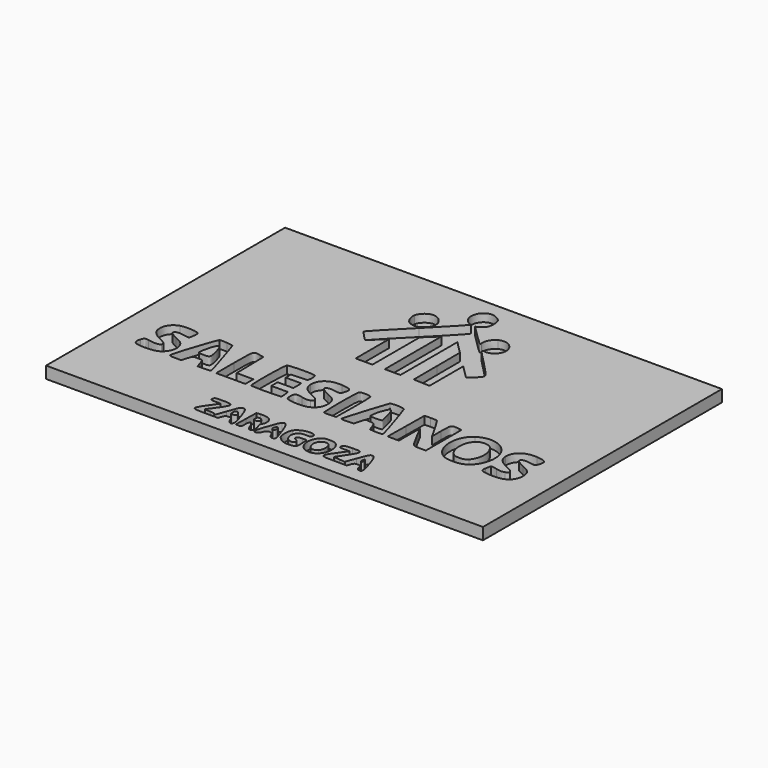
from build123d import *

# Parameters (mm, degrees)
F1_W     = 111
F1_H     = 75.8981681683
F2_DEPTH = 1
F0_W     = 111
F0_H     = 75.8981681683
F3_DEPTH = 3


# Not quite as in the source:
# - ends of sketch curves that miss each other by under 0.0002 mm in the source are joined
# - a feature names something its author has since deleted; it is built from what else it names


with BuildPart() as f2:
    # F1 (on Top) → F2 (new body)
    with BuildSketch(Plane.XY):
        Rectangle(F1_W, F1_H)
    extrude(amount=F2_DEPTH)

    # F0 (on Top) → F3 (join)
    with BuildSketch(Plane.XY):
        Rectangle(F0_W, F0_H)
        with BuildLine():
            add(Edge.make_bspline(
                [(-11.3553504545, -34.4155459636), (-11.5365297, -34.4751549818), (-11.8889547, -34.2324080727), (-12.1385170091, -33.8761071545)],
                knots=[0, 0, 0, 0, 1, 1, 1, 1], degree=3))
            add(Edge.make_bspline(
                [(-12.1385170091, -33.8761071545), (-12.3880803273, -33.5198062364), (-12.5922668455, -33.0645720273), (-12.5922668455, -32.8644723273)],
                knots=[0, 0, 0, 0, 1, 1, 1, 1], degree=3))
            add(Edge.make_bspline(
                [(-12.5922668455, -32.8644723273), (-12.5922668455, -32.6528175273), (-12.9379400182, -32.5006587273), (-13.4187698182, -32.5006587273)],
                knots=[0, 0, 0, 0, 1, 1, 1, 1], degree=3))
            add(Edge.make_bspline(
                [(-13.4187698182, -32.5006587273), (-14.0810664545, -32.5006587273), (-14.3044489091, -32.6704029545), (-14.5431100091, -33.3550216909)],
                knots=[0, 0, 0, 0, 1, 1, 1, 1], degree=3))
            Line((-14.5431100091, -33.3550216909), (-14.8409411727, -34.2093856636))
            Line((-14.8409411727, -34.2093856636), (-17.9884218545, -34.2093856636))
            add(Edge.make_bspline(
                [(-17.9884218545, -34.2093856636), (-21.7751353909, -34.2093856636), (-21.7852283182, -34.1913865091), (-19.6949197091, -31.1676597273)],
                knots=[0, 0, 0, 0, 1, 1, 1, 1], degree=3))
            Line((-19.6949197091, -31.1676597273), (-18.2539358727, -29.0832038455))
            Line((-18.2539358727, -29.0832038455), (-19.5723323182, -29.0832038455))
            add(Edge.make_bspline(
                [(-19.5723323182, -29.0832038455), (-20.7766661727, -29.0832038455), (-20.8828578545, -29.0277643909), (-20.7997259182, -28.4424311182)],
                knots=[0, 0, 0, 0, 1, 1, 1, 1], degree=3))
            add(Edge.make_bspline(
                [(-20.7997259182, -28.4424311182), (-20.7146050636, -27.8430916636), (-20.5708610727, -27.8016583909), (-18.5767137818, -27.8016583909)],
                knots=[0, 0, 0, 0, 1, 1, 1, 1], degree=3))
            add(Edge.make_bspline(
                [(-18.5767137818, -27.8016583909), (-15.8485941273, -27.8016583909), (-15.7638496636, -28.1012090455), (-17.7110812909, -30.8614874182)],
                knots=[0, 0, 0, 0, 1, 1, 1, 1], degree=3))
            Line((-17.7110812909, -30.8614874182), (-19.1687827364, -32.9278402091))
            Line((-19.1687827364, -32.9278402091), (-17.7316455545, -33.0139197))
            add(Edge.make_bspline(
                [(-17.7316455545, -33.0139197), (-16.6065747818, -33.0813098182), (-16.2931309636, -33.2049870273), (-16.2881591727, -33.5834960182)],
                knots=[0, 0, 0, 0, 1, 1, 1, 1], degree=3))
            add(Edge.make_bspline(
                [(-16.2881591727, -33.5834960182), (-16.2846556091, -33.8494197273), (-15.8040871636, -32.6572918364), (-15.2202039545, -30.9343246091)],
                knots=[0, 0, 0, 0, 1, 1, 1, 1], degree=3))
            add(Edge.make_bspline(
                [(-15.2202039545, -30.9343246091), (-14.2654788273, -28.1170437), (-14.0900635091, -27.8016583909), (-13.4778409909, -27.8016583909)],
                knots=[0, 0, 0, 0, 1, 1, 1, 1], degree=3))
            add(Edge.make_bspline(
                [(-13.4778409909, -27.8016583909), (-12.8766417818, -27.8016583909), (-12.6837490091, -28.1156794091), (-11.8273920818, -30.4885203545)],
                knots=[0, 0, 0, 0, 1, 1, 1, 1], degree=3))
            add(Edge.make_bspline(
                [(-11.8273920818, -30.4885203545), (-10.8589251545, -33.1719968182), (-10.7340208909, -34.2111253364), (-11.3553504545, -34.4155459636)],
                knots=[0, 0, 0, 0, 1, 1, 1, 1], degree=3))
        make_face(mode=Mode.SUBTRACT)
        with BuildLine():
            Line((-10.3326176455, -34.2093856636), (-10.2520942091, -31.0055220273))
            Line((-10.2520942091, -31.0055220273), (-10.1715697636, -27.8016583909))
            Line((-10.1715697636, -27.8016583909), (-9.2066033727, -27.7094779364))
            add(Edge.make_bspline(
                [(-9.2066033727, -27.7094779364), (-7.9795922182, -27.5922679909), (-7.0573345909, -27.8239118727), (-6.4892426455, -28.3920038182)],
                knots=[0, 0, 0, 0, 1, 1, 1, 1], degree=3))
            add(Edge.make_bspline(
                [(-6.4892426455, -28.3920038182), (-5.9702197636, -28.9110267), (-5.8971060818, -30.2481882), (-6.3623161636, -30.7133982818)],
                knots=[0, 0, 0, 0, 1, 1, 1, 1], degree=3))
            add(Edge.make_bspline(
                [(-6.3623161636, -30.7133982818), (-6.5993475818, -30.9504297), (-6.5993475818, -31.2720491727), (-6.3623161636, -31.9520028818)],
                knots=[0, 0, 0, 0, 1, 1, 1, 1], degree=3))
            add(Edge.make_bspline(
                [(-6.3623161636, -31.9520028818), (-6.1862227364, -32.4571426909), (-6.0421457455, -33.1717041818), (-6.0421457455, -33.5399123727)],
                knots=[0, 0, 0, 0, 1, 1, 1, 1], degree=3))
            add(Edge.make_bspline(
                [(-6.0421457455, -33.5399123727), (-6.0421457455, -34.5283562727), (-7.1124894818, -34.4433070636), (-7.4729629909, -33.4262191091)],
                knots=[0, 0, 0, 0, 1, 1, 1, 1], degree=3))
            add(Edge.make_bspline(
                [(-7.4729629909, -33.4262191091), (-8.2103047091, -31.3457925273), (-8.8900243091, -31.0953492818), (-8.8900243091, -32.9041084091)],
                knots=[0, 0, 0, 0, 1, 1, 1, 1], degree=3))
            add(Edge.make_bspline(
                [(-8.8900243091, -32.9041084091), (-8.8900243091, -34.1110457182), (-8.9443678909, -34.2093856636), (-9.6113214818, -34.2093856636)],
                knots=[0, 0, 0, 0, 1, 1, 1, 1], degree=3))
            Line((-9.6113214818, -34.2093856636), (-10.3326176455, -34.2093856636))
        make_face(mode=Mode.SUBTRACT)
        with BuildLine():
            add(Edge.make_bspline(
                [(-4.081359, -33.3264916636), (-4.3966989, -34.2310780909), (-5.4122066182, -34.6980611455), (-5.6599636636, -34.0524185455)],
                knots=[0, 0, 0, 0, 1, 1, 1, 1], degree=3))
            add(Edge.make_bspline(
                [(-5.6599636636, -34.0524185455), (-5.8610835545, -33.5283068182), (-4.0886718818, -28.3318135636), (-3.5587952182, -27.8920557818)],
                knots=[0, 0, 0, 0, 1, 1, 1, 1], degree=3))
            add(Edge.make_bspline(
                [(-3.5587952182, -27.8920557818), (-2.8344657273, -27.2909140909), (-2.2841247, -28.0040457), (-1.3082682, -30.8082861273)],
                knots=[0, 0, 0, 0, 1, 1, 1, 1], degree=3))
            add(Edge.make_bspline(
                [(-1.3082682, -30.8082861273), (-0.1767432818, -34.0598515091), (-0.1645312636, -34.2093856636), (-1.0304967545, -34.2093856636)],
                knots=[0, 0, 0, 0, 1, 1, 1, 1], degree=3))
            add(Edge.make_bspline(
                [(-1.0304967545, -34.2093856636), (-1.5345770182, -34.2093856636), (-1.7929880455, -33.9845511273), (-2.0124431182, -33.3550216909)],
                knots=[0, 0, 0, 0, 1, 1, 1, 1], degree=3))
            add(Edge.make_bspline(
                [(-2.0124431182, -33.3550216909), (-2.4296568, -32.1581974909), (-3.6681342545, -32.1411196364), (-4.081359, -33.3264916636)],
                knots=[0, 0, 0, 0, 1, 1, 1, 1], degree=3))
        make_face(mode=Mode.SUBTRACT)
        with BuildLine():
            add(Edge.make_bspline(
                [(-42.0060337364, -19.2096196364), (-42.9500251636, -19.6575712364), (-45.3833419364, -19.7937904364), (-46.9597225636, -19.4869289182)],
                knots=[0, 0, 0, 0, 1, 1, 1, 1], degree=3))
            add(Edge.make_bspline(
                [(-46.9597225636, -19.4869289182), (-48.0138643364, -19.2817272545), (-48.2886367636, -18.7088058), (-47.8990519909, -17.5283510727)],
                knots=[0, 0, 0, 0, 1, 1, 1, 1], degree=3))
            add(Edge.make_bspline(
                [(-47.8990519909, -17.5283510727), (-47.5662205091, -16.5198636), (-47.5247781545, -16.4950984909), (-46.5205853727, -16.7045686091)],
                knots=[0, 0, 0, 0, 1, 1, 1, 1], degree=3))
            add(Edge.make_bspline(
                [(-46.5205853727, -16.7045686091), (-44.9145808636, -17.0395756909), (-43.6095346909, -16.9735105091), (-43.3439328818, -16.5437598818)],
                knots=[0, 0, 0, 0, 1, 1, 1, 1], degree=3))
            add(Edge.make_bspline(
                [(-43.3439328818, -16.5437598818), (-42.9966027818, -15.9817648636), (-43.1955238636, -15.7840284545), (-45.0498979364, -14.8479422455)],
                knots=[0, 0, 0, 0, 1, 1, 1, 1], degree=3))
            add(Edge.make_bspline(
                [(-45.0498979364, -14.8479422455), (-47.1731503364, -13.7761282636), (-47.9059642636, -12.8574286909), (-47.9059642636, -11.2674061636)],
                knots=[0, 0, 0, 0, 1, 1, 1, 1], degree=3))
            add(Edge.make_bspline(
                [(-47.9059642636, -11.2674061636), (-47.9059642636, -9.7685731636), (-46.9405306636, -8.4891811091), (-45.4344271636, -7.9921210909)],
                knots=[0, 0, 0, 0, 1, 1, 1, 1], degree=3))
            add(Edge.make_bspline(
                [(-45.4344271636, -7.9921210909), (-44.3034774273, -7.6188755182), (-41.1813158455, -7.7847246545), (-40.7236820182, -8.2423584818)],
                knots=[0, 0, 0, 0, 1, 1, 1, 1], degree=3))
            add(Edge.make_bspline(
                [(-40.7236820182, -8.2423584818), (-40.5603879, -8.4056526), (-40.5263724545, -9.0221476091), (-40.6426772455, -9.7105423636)],
                knots=[0, 0, 0, 0, 1, 1, 1, 1], degree=3))
            Line((-40.6426772455, -9.7105423636), (-40.8431644364, -10.8972302455))
            Line((-40.8431644364, -10.8972302455), (-42.0250662, -10.6883585182))
            add(Edge.make_bspline(
                [(-42.0250662, -10.6883585182), (-43.4975901818, -10.4281250727), (-44.2100093727, -10.4643645545), (-44.5631094545, -10.8174646364)],
                knots=[0, 0, 0, 0, 1, 1, 1, 1], degree=3))
            add(Edge.make_bspline(
                [(-44.5631094545, -10.8174646364), (-44.9928943909, -11.2472495727), (-44.5569015273, -11.6855572909), (-42.9671898, -12.4218283636)],
                knots=[0, 0, 0, 0, 1, 1, 1, 1], degree=3))
            add(Edge.make_bspline(
                [(-42.9671898, -12.4218283636), (-42.1592662091, -12.7960164273), (-41.2948981091, -13.2697704818), (-41.0463751636, -13.4746119)],
                knots=[0, 0, 0, 0, 1, 1, 1, 1], degree=3))
            add(Edge.make_bspline(
                [(-41.0463751636, -13.4746119), (-39.2149609364, -14.9841271364), (-39.7422745091, -18.1353939273), (-42.0060337364, -19.2096196364)],
                knots=[0, 0, 0, 0, 1, 1, 1, 1], degree=3))
        make_face(mode=Mode.SUBTRACT)
        with BuildLine():
            add(Edge.make_bspline(
                [(-37.5612062455, -19.4004155182), (-38.7397729636, -19.4004155182), (-39.0775399091, -19.3022632636), (-39.0775399091, -18.9597838636)],
                knots=[0, 0, 0, 0, 1, 1, 1, 1], degree=3))
            add(Edge.make_bspline(
                [(-39.0775399091, -18.9597838636), (-39.0775399091, -17.9400753), (-35.8349251636, -8.0276481545), (-35.4534686182, -7.8812704364)],
                knots=[0, 0, 0, 0, 1, 1, 1, 1], degree=3))
            add(Edge.make_bspline(
                [(-35.4534686182, -7.8812704364), (-35.2287682909, -7.7950416), (-34.3552104, -7.8055563273), (-33.5122289727, -7.9046228182)],
                knots=[0, 0, 0, 0, 1, 1, 1, 1], degree=3))
            Line((-33.5122289727, -7.9046228182), (-31.9795349182, -8.0847596727))
            Line((-31.9795349182, -8.0847596727), (-31.1347462091, -10.6811142545))
            add(Edge.make_bspline(
                [(-31.1347462091, -10.6811142545), (-29.9778497182, -14.2366844182), (-28.5403886182, -18.9568383273), (-28.5403886182, -19.2001442727)],
                knots=[0, 0, 0, 0, 1, 1, 1, 1], degree=3))
            add(Edge.make_bspline(
                [(-28.5403886182, -19.2001442727), (-28.5403886182, -19.3102946182), (-29.2868141727, -19.4004155182), (-30.1991151, -19.4004155182)],
                knots=[0, 0, 0, 0, 1, 1, 1, 1], degree=3))
            Line((-30.1991151, -19.4004155182), (-31.8578456182, -19.4004155182))
            Line((-31.8578456182, -19.4004155182), (-32.2779412636, -18.0476736545))
            add(Edge.make_bspline(
                [(-32.2779412636, -18.0476736545), (-32.6957079273, -16.7024323636), (-32.7049865182, -16.6949307818), (-33.9513580909, -16.6949307818)],
                knots=[0, 0, 0, 0, 1, 1, 1, 1], degree=3))
            add(Edge.make_bspline(
                [(-33.9513580909, -16.6949307818), (-35.1977296636, -16.6949307818), (-35.2070072455, -16.7024212636), (-35.6247739091, -18.0476736545)],
                knots=[0, 0, 0, 0, 1, 1, 1, 1], degree=3))
            Line((-35.6247739091, -18.0476736545), (-36.0448735909, -19.4004155182))
            Line((-36.0448735909, -19.4004155182), (-37.5612062455, -19.4004155182))
        make_face(mode=Mode.SUBTRACT)
        with BuildLine():
            Line((-27.1164493364, -19.4004155182), (-27.1164493364, -13.6957218818))
            add(Edge.make_bspline(
                [(-27.1164493364, -13.6957218818), (-27.1164493364, -7.3469991818), (-27.1530157636, -7.4570899909), (-25.1976417818, -7.9189509)],
                knots=[0, 0, 0, 0, 1, 1, 1, 1], degree=3))
            Line((-25.1976417818, -7.9189509), (-24.1261759364, -8.1720329182))
            Line((-24.1261759364, -8.1720329182), (-24.0475606909, -12.5046787636))
            Line((-24.0475606909, -12.5046787636), (-23.9689474636, -16.8373246091))
            Line((-23.9689474636, -16.8373246091), (-21.8404548545, -16.8373246091))
            Line((-21.8404548545, -16.8373246091), (-19.7119642636, -16.8373246091))
            Line((-19.7119642636, -16.8373246091), (-19.7119642636, -18.1188700636))
            Line((-19.7119642636, -18.1188700636), (-19.7119642636, -19.4004155182))
            Line((-19.7119642636, -19.4004155182), (-23.4142068, -19.4004155182))
            Line((-23.4142068, -19.4004155182), (-27.1164493364, -19.4004155182))
        make_face(mode=Mode.SUBTRACT)
        with BuildLine():
            add(Edge.make_bspline(
                [(-10.7686448182, -19.1601116182), (-10.9430429727, -19.4422968273), (-18.1037811273, -19.4897362091), (-18.3829582364, -19.2105560727)],
                knots=[0, 0, 0, 0, 1, 1, 1, 1], degree=3))
            add(Edge.make_bspline(
                [(-18.3829582364, -19.2105560727), (-18.7421582727, -18.8513530091), (-18.6001973455, -8.4349888909), (-18.2310668455, -8.0658583909)],
                knots=[0, 0, 0, 0, 1, 1, 1, 1], degree=3))
            add(Edge.make_bspline(
                [(-18.2310668455, -8.0658583909), (-17.8347907909, -7.6695813273), (-11.8234596545, -7.5882970364), (-11.2198174364, -7.9710522818)],
                knots=[0, 0, 0, 0, 1, 1, 1, 1], degree=3))
            add(Edge.make_bspline(
                [(-11.2198174364, -7.9710522818), (-10.9844086364, -8.1203180182), (-10.8780686182, -8.6238089727), (-10.9350297818, -9.3194348727)],
                knots=[0, 0, 0, 0, 1, 1, 1, 1], degree=3))
            Line((-10.9350297818, -9.3194348727), (-11.0259337364, -10.4295973364))
            Line((-11.0259337364, -10.4295973364), (-13.0906457455, -10.5132711545))
            Line((-13.0906457455, -10.5132711545), (-15.1553577545, -10.5969449727))
            Line((-15.1553577545, -10.5969449727), (-15.1553577545, -11.4388315364))
            Line((-15.1553577545, -11.4388315364), (-15.1553577545, -12.2807191091))
            Line((-15.1553577545, -12.2807191091), (-13.1618431636, -12.2807191091))
            Line((-13.1618431636, -12.2807191091), (-11.1683275636, -12.2807191091))
            Line((-11.1683275636, -12.2807191091), (-11.1683275636, -13.5622645636))
            Line((-11.1683275636, -13.5622645636), (-11.1683275636, -14.8438100182))
            Line((-11.1683275636, -14.8438100182), (-13.1618431636, -14.8438100182))
            Line((-13.1618431636, -14.8438100182), (-15.1553577545, -14.8438100182))
            Line((-15.1553577545, -14.8438100182), (-15.1553577545, -15.8405678182))
            Line((-15.1553577545, -15.8405678182), (-15.1553577545, -16.8373246091))
            Line((-15.1553577545, -16.8373246091), (-13.0567100182, -16.8373246091))
            Line((-13.0567100182, -16.8373246091), (-10.9580632909, -16.8373246091))
            Line((-10.9580632909, -16.8373246091), (-10.7890930364, -17.8785661636))
            add(Edge.make_bspline(
                [(-10.7890930364, -17.8785661636), (-10.6961608091, -18.4512525), (-10.6869568909, -19.0279479545), (-10.7686448182, -19.1601116182)],
                knots=[0, 0, 0, 0, 1, 1, 1, 1], degree=3))
        make_face(mode=Mode.SUBTRACT)
        with BuildLine():
            add(Edge.make_bspline(
                [(-3.6601170273, -19.2925326), (-4.7367383182, -19.7423722091), (-7.5199381909, -19.7765894727), (-8.6764340727, -19.3542001636)],
                knots=[0, 0, 0, 0, 1, 1, 1, 1], degree=3))
            add(Edge.make_bspline(
                [(-8.6764340727, -19.3542001636), (-9.30735, -19.1237702182), (-9.4587519818, -18.8928438), (-9.4552403455, -18.1663356818)],
                knots=[0, 0, 0, 0, 1, 1, 1, 1], degree=3))
            add(Edge.make_bspline(
                [(-9.4552403455, -18.1663356818), (-9.4476075818, -16.5868480636), (-9.1572386455, -16.3974639), (-7.3923336, -16.8208582636)],
                knots=[0, 0, 0, 0, 1, 1, 1, 1], degree=3))
            add(Edge.make_bspline(
                [(-7.3923336, -16.8208582636), (-6.2100685636, -17.1044784), (-5.7048712364, -17.1140647636), (-5.233539, -16.8618142364)],
                knots=[0, 0, 0, 0, 1, 1, 1, 1], degree=3))
            add(Edge.make_bspline(
                [(-5.233539, -16.8618142364), (-4.1449115455, -16.2791974364), (-4.5131762455, -15.7128340636), (-6.5470978636, -14.8416566182)],
                knots=[0, 0, 0, 0, 1, 1, 1, 1], degree=3))
            add(Edge.make_bspline(
                [(-6.5470978636, -14.8416566182), (-8.4610315091, -14.0218752), (-9.4599507818, -12.8670059727), (-9.4585350273, -11.4757006909)],
                knots=[0, 0, 0, 0, 1, 1, 1, 1], degree=3))
            add(Edge.make_bspline(
                [(-9.4585350273, -11.4757006909), (-9.4559719364, -9.0022039364), (-7.4633342455, -7.5549122727), (-4.3989229364, -7.8008943273)],
                knots=[0, 0, 0, 0, 1, 1, 1, 1], degree=3))
            add(Edge.make_bspline(
                [(-4.3989229364, -7.8008943273), (-2.0766848727, -7.9873026818), (-1.6656619636, -8.3485249364), (-2.1139102364, -9.8090538545)],
                knots=[0, 0, 0, 0, 1, 1, 1, 1], degree=3))
            add(Edge.make_bspline(
                [(-2.1139102364, -9.8090538545), (-2.4429707455, -10.8812260636), (-2.4537276545, -10.8875480182), (-3.6029833091, -10.6842545455)],
                knots=[0, 0, 0, 0, 1, 1, 1, 1], degree=3))
            add(Edge.make_bspline(
                [(-3.6029833091, -10.6842545455), (-5.0516140364, -10.4280090273), (-5.7650988273, -10.4658166364), (-6.1167458182, -10.8174646364)],
                knots=[0, 0, 0, 0, 1, 1, 1, 1], degree=3))
            add(Edge.make_bspline(
                [(-6.1167458182, -10.8174646364), (-6.5633442273, -11.2640630455), (-6.1060383545, -11.6764986818), (-4.2121048909, -12.5352542182)],
                knots=[0, 0, 0, 0, 1, 1, 1, 1], degree=3))
            add(Edge.make_bspline(
                [(-4.2121048909, -12.5352542182), (-2.0595777545, -13.511253), (-1.4855402455, -14.2423746818), (-1.4855402455, -16.0079225182)],
                knots=[0, 0, 0, 0, 1, 1, 1, 1], degree=3))
            add(Edge.make_bspline(
                [(-1.4855402455, -16.0079225182), (-1.4855402455, -17.5672424455), (-2.2329970909, -18.6962436273), (-3.6601170273, -19.2925326)],
                knots=[0, 0, 0, 0, 1, 1, 1, 1], degree=3))
        make_face(mode=Mode.SUBTRACT)
        with BuildLine():
            add(Edge.make_bspline(
                [(4.8672834, -33.9506840182), (4.3306034455, -34.4865778909), (2.3567782364, -34.5194823273), (1.3663000091, -34.0090458)],
                knots=[0, 0, 0, 0, 1, 1, 1, 1], degree=3))
            add(Edge.make_bspline(
                [(1.3663000091, -34.0090458), (0.8202627545, -33.7276497), (0.2134197, -33.1770291545), (0.0177559636, -32.7854463818)],
                knots=[0, 0, 0, 0, 1, 1, 1, 1], degree=3))
            add(Edge.make_bspline(
                [(0.0177559636, -32.7854463818), (-0.4760325818, -31.7972123727), (-0.4342824545, -29.9049994091), (0.0980806091, -29.1449430545)],
                knots=[0, 0, 0, 0, 1, 1, 1, 1], degree=3))
            add(Edge.make_bspline(
                [(0.0980806091, -29.1449430545), (1.2483695727, -27.5026798909), (4.7797932, -27.0494568), (4.7797932, -28.5440970273)],
                knots=[0, 0, 0, 0, 1, 1, 1, 1], degree=3))
            add(Edge.make_bspline(
                [(4.7797932, -28.5440970273), (4.7797932, -29.0003413364), (4.5634148455, -29.0832038455), (3.3720013909, -29.0832038455)],
                knots=[0, 0, 0, 0, 1, 1, 1, 1], degree=3))
            add(Edge.make_bspline(
                [(3.3720013909, -29.0832038455), (2.2400728364, -29.0832038455), (1.8773409818, -29.2072312091), (1.5208806273, -29.7161480455)],
                knots=[0, 0, 0, 0, 1, 1, 1, 1], degree=3))
            add(Edge.make_bspline(
                [(1.5208806273, -29.7161480455), (0.5511694909, -31.1006036182), (1.3778712545, -33.0702340364), (2.9286724364, -33.0702340364)],
                knots=[0, 0, 0, 0, 1, 1, 1, 1], degree=3))
            add(Edge.make_bspline(
                [(2.9286724364, -33.0702340364), (3.8298380455, -33.0702340364), (3.9254443636, -32.0719898455), (3.0462981273, -31.8420886636)],
                knots=[0, 0, 0, 0, 1, 1, 1, 1], degree=3))
            add(Edge.make_bspline(
                [(3.0462981273, -31.8420886636), (2.6611281273, -31.7413652455), (2.4871003091, -31.5041572364), (2.5518183545, -31.1681017091)],
                knots=[0, 0, 0, 0, 1, 1, 1, 1], degree=3))
            add(Edge.make_bspline(
                [(2.5518183545, -31.1681017091), (2.6284921091, -30.7699679182), (2.9153332636, -30.6495369545), (3.7869375545, -30.6495369545)],
                knots=[0, 0, 0, 0, 1, 1, 1, 1], degree=3))
            Line((3.7869375545, -30.6495369545), (4.9221870273, -30.6495369545))
            Line((4.9221870273, -30.6495369545), (5.0096772273, -32.185338))
            add(Edge.make_bspline(
                [(5.0096772273, -32.185338), (5.0577977455, -33.0300278182), (4.9937295545, -33.8244346364), (4.8672834, -33.9506840182)],
                knots=[0, 0, 0, 0, 1, 1, 1, 1], degree=3))
        make_face(mode=Mode.SUBTRACT)
        with BuildLine():
            add(Edge.make_bspline(
                [(10.5467477455, -33.3512365909), (9.5478718636, -34.4475502909), (8.3566612364, -34.6719065182), (7.0651621091, -34.0069670727)],
                knots=[0, 0, 0, 0, 1, 1, 1, 1], degree=3))
            add(Edge.make_bspline(
                [(7.0651621091, -34.0069670727), (5.2252079455, -33.0596517), (4.8539926636, -30.3067487727), (6.3341625273, -28.5859470545)],
                knots=[0, 0, 0, 0, 1, 1, 1, 1], degree=3))
            add(Edge.make_bspline(
                [(6.3341625273, -28.5859470545), (6.9086258727, -27.9180963818), (7.2275056636, -27.8016583909), (8.4820357364, -27.8016583909)],
                knots=[0, 0, 0, 0, 1, 1, 1, 1], degree=3))
            add(Edge.make_bspline(
                [(8.4820357364, -27.8016583909), (9.7431531545, -27.8016583909), (10.0542589091, -27.9167149364), (10.6426023, -28.6007050091)],
                knots=[0, 0, 0, 0, 1, 1, 1, 1], degree=3))
            add(Edge.make_bspline(
                [(10.6426023, -28.6007050091), (11.6729164091, -29.7985171091), (11.6251117364, -32.1676789091), (10.5467477455, -33.3512365909)],
                knots=[0, 0, 0, 0, 1, 1, 1, 1], degree=3))
        make_face(mode=Mode.SUBTRACT)
        with BuildLine():
            add(Edge.make_bspline(
                [(21.0134291727, -30.9365718545), (21.9769263273, -33.9176635364), (21.9674196818, -34.5173410364), (20.9603439273, -34.285347)],
                knots=[0, 0, 0, 0, 1, 1, 1, 1], degree=3))
            add(Edge.make_bspline(
                [(20.9603439273, -34.285347), (20.6965968273, -34.2245876182), (20.3980673727, -33.7981770818), (20.2969423364, -33.3377662364)],
                knots=[0, 0, 0, 0, 1, 1, 1, 1], degree=3))
            add(Edge.make_bspline(
                [(20.2969423364, -33.3377662364), (20.1464576182, -32.6526126818), (19.9671613364, -32.5006587273), (19.3092068182, -32.5006587273)],
                knots=[0, 0, 0, 0, 1, 1, 1, 1], degree=3))
            add(Edge.make_bspline(
                [(19.3092068182, -32.5006587273), (18.6720537, -32.5006587273), (18.4435602, -32.6778530727), (18.2074965, -33.3550216909)],
                knots=[0, 0, 0, 0, 1, 1, 1, 1], degree=3))
            Line((18.2074965, -33.3550216909), (17.9096653364, -34.2093856636))
            Line((17.9096653364, -34.2093856636), (14.7621836455, -34.2093856636))
            add(Edge.make_bspline(
                [(14.7621836455, -34.2093856636), (10.9602399, -34.2093856636), (10.9236623727, -34.1435656909), (13.0460610818, -31.1213818091)],
                knots=[0, 0, 0, 0, 1, 1, 1, 1], degree=3))
            Line((13.0460610818, -31.1213818091), (14.4774161727, -29.0832038455))
            Line((14.4774161727, -29.0832038455), (13.1686444364, -29.0832038455))
            add(Edge.make_bspline(
                [(13.1686444364, -29.0832038455), (11.9742985636, -29.0832038455), (11.8678334182, -29.0271831545), (11.9508805909, -28.4424311182)],
                knots=[0, 0, 0, 0, 1, 1, 1, 1], degree=3))
            add(Edge.make_bspline(
                [(11.9508805909, -28.4424311182), (12.0344091, -27.8542986273), (12.2118426, -27.7947774), (14.1107145545, -27.7179018273)],
                knots=[0, 0, 0, 0, 1, 1, 1, 1], degree=3))
            add(Edge.make_bspline(
                [(14.1107145545, -27.7179018273), (16.8515013273, -27.6069401727), (16.9430692636, -27.8948156455), (15.0684134727, -30.7287142636)],
                knots=[0, 0, 0, 0, 1, 1, 1, 1], degree=3))
            Line((15.0684134727, -30.7287142636), (13.6136686636, -32.9278402091))
            Line((13.6136686636, -32.9278402091), (15.1060798091, -33.0702340364))
            Line((15.1060798091, -33.0702340364), (16.5984909545, -33.2126278636))
            Line((16.5984909545, -33.2126278636), (17.5364308636, -30.6513967091))
            add(Edge.make_bspline(
                [(17.5364308636, -30.6513967091), (18.5974334455, -27.7541160818), (18.7475770909, -27.5346751364), (19.5045516818, -27.7749306)],
                knots=[0, 0, 0, 0, 1, 1, 1, 1], degree=3))
            add(Edge.make_bspline(
                [(19.5045516818, -27.7749306), (19.8976127727, -27.8996824909), (20.3136478364, -28.7714240182), (21.0134291727, -30.9365718545)],
                knots=[0, 0, 0, 0, 1, 1, 1, 1], degree=3))
        make_face(mode=Mode.SUBTRACT)
        with BuildLine():
            add(Edge.make_bspline(
                [(1.7785822636, -19.3420113545), (0.9893974909, -19.3882065273), (0.2525088545, -19.3348064455), (0.1410517364, -19.2233493273)],
                knots=[0, 0, 0, 0, 1, 1, 1, 1], degree=3))
            add(Edge.make_bspline(
                [(0.1410517364, -19.2233493273), (0.0295915909, -19.1118912), (-0.0615999545, -16.6228140818), (-0.0615999545, -13.6920649364)],
                knots=[0, 0, 0, 0, 1, 1, 1, 1], degree=3))
            add(Edge.make_bspline(
                [(-0.0615999545, -13.6920649364), (-0.0615999545, -9.7551855545), (0.0320830364, -8.2856807727), (0.2970844364, -8.0657473909)],
                knots=[0, 0, 0, 0, 1, 1, 1, 1], degree=3))
            add(Edge.make_bspline(
                [(0.2970844364, -8.0657473909), (0.7040830909, -7.7279683364), (2.7342337364, -7.8429401182), (3.1167235909, -8.2254309818)],
                knots=[0, 0, 0, 0, 1, 1, 1, 1], degree=3))
            add(Edge.make_bspline(
                [(3.1167235909, -8.2254309818), (3.2553605727, -8.3640679636), (3.3338426182, -10.9031172818), (3.2911278, -13.8677617909)],
                knots=[0, 0, 0, 0, 1, 1, 1, 1], degree=3))
            Line((3.2911278, -13.8677617909), (3.2134600909, -19.2580216909))
            Line((3.2134600909, -19.2580216909), (1.7785822636, -19.3420113545))
        make_face(mode=Mode.SUBTRACT)
        with BuildLine():
            add(Edge.make_bspline(
                [(6.1039061455, -19.3434301364), (5.2070665091, -19.3910410636), (4.4950055455, -19.3079000455), (4.4950055455, -19.1555777727)],
                knots=[0, 0, 0, 0, 1, 1, 1, 1], degree=3))
            add(Edge.make_bspline(
                [(4.4950055455, -19.1555777727), (4.4950055455, -18.6306850091), (7.6846783364, -8.4332744455), (7.9500460364, -8.1097810909)],
                knots=[0, 0, 0, 0, 1, 1, 1, 1], degree=3))
            add(Edge.make_bspline(
                [(7.9500460364, -8.1097810909), (8.2585745727, -7.7336787818), (11.2335340091, -7.7926096909), (11.6059107545, -8.1821995091)],
                knots=[0, 0, 0, 0, 1, 1, 1, 1], degree=3))
            add(Edge.make_bspline(
                [(11.6059107545, -8.1821995091), (11.8817316273, -8.4707722636), (15.0321568364, -18.4605109091), (15.0321568364, -19.0465444909)],
                knots=[0, 0, 0, 0, 1, 1, 1, 1], degree=3))
            add(Edge.make_bspline(
                [(15.0321568364, -19.0465444909), (15.0321568364, -19.3311979364), (14.6233297091, -19.4070260727), (13.4314581273, -19.3434301364)],
                knots=[0, 0, 0, 0, 1, 1, 1, 1], degree=3))
            Line((13.4314581273, -19.3434301364), (11.8307624455, -19.2580216909))
            Line((11.8307624455, -19.2580216909), (11.3602304182, -17.9764762364))
            add(Edge.make_bspline(
                [(11.3602304182, -17.9764762364), (10.9151184, -16.7641624909), (10.8253789364, -16.6902344727), (9.6990710182, -16.6080056727)],
                knots=[0, 0, 0, 0, 1, 1, 1, 1], degree=3))
            Line((9.6990710182, -16.6080056727), (8.5084446545, -16.5210795545))
            Line((8.5084446545, -16.5210795545), (8.1106267091, -17.8895511273))
            Line((8.1106267091, -17.8895511273), (7.7128097727, -19.2580216909))
            Line((7.7128097727, -19.2580216909), (6.1039061455, -19.3434301364))
        make_face(mode=Mode.SUBTRACT)
        with BuildLine():
            Line((16.4443149818, -19.4004155182), (16.5214065, -13.6382824091))
            Line((16.5214065, -13.6382824091), (16.5984909545, -7.8761472818))
            Line((16.5984909545, -7.8761472818), (18.0792622364, -7.8456434727))
            add(Edge.make_bspline(
                [(18.0792622364, -7.8456434727), (18.8936874, -7.8288693545), (19.6720809545, -7.8907730455), (19.8090267, -7.9832158636)],
                knots=[0, 0, 0, 0, 1, 1, 1, 1], degree=3))
            add(Edge.make_bspline(
                [(19.8090267, -7.9832158636), (19.9459694182, -8.0756607), (20.7842232545, -9.4328405455), (21.6718095273, -10.9991736545)],
                knots=[0, 0, 0, 0, 1, 1, 1, 1], degree=3))
            Line((21.6718095273, -10.9991736545), (23.2856001818, -13.8470522182))
            Line((23.2856001818, -13.8470522182), (23.2881632727, -10.9477836818))
            add(Edge.make_bspline(
                [(23.2881632727, -10.9477836818), (23.2911542182, -7.7511764182), (23.3304340909, -7.6945401818), (25.3555786364, -7.9678514455)],
                knots=[0, 0, 0, 0, 1, 1, 1, 1], degree=3))
            Line((25.3555786364, -7.9678514455), (26.1387451909, -8.0735476636))
            Line((26.1387451909, -8.0735476636), (26.1387451909, -13.7369815909))
            Line((26.1387451909, -13.7369815909), (26.1387451909, -19.4004155182))
            Line((26.1387451909, -19.4004155182), (24.6072812182, -19.4004155182))
            add(Edge.make_bspline(
                [(24.6072812182, -19.4004155182), (23.7274770545, -19.4004155182), (22.9517525455, -19.2489398727), (22.7842454727, -19.0444314545)],
                knots=[0, 0, 0, 0, 1, 1, 1, 1], degree=3))
            add(Edge.make_bspline(
                [(22.7842454727, -19.0444314545), (22.6238787273, -18.8486395636), (21.7771243091, -17.3428236545), (20.9025724636, -15.6981729818)],
                knots=[0, 0, 0, 0, 1, 1, 1, 1], degree=3))
            Line((20.9025724636, -15.6981729818), (19.3124732455, -12.7079005909))
            Line((19.3124732455, -12.7079005909), (19.3081442455, -16.0541580545))
            Line((19.3081442455, -16.0541580545), (19.3039867909, -19.4004155182))
            Line((19.3039867909, -19.4004155182), (17.8741493727, -19.4004155182))
            Line((17.8741493727, -19.4004155182), (16.4443149818, -19.4004155182))
        make_face(mode=Mode.SUBTRACT)
        with BuildLine():
            add(Edge.make_bspline(
                [(35.6216770091, -19.3004438727), (34.4609469818, -19.7854260818), (31.9589060727, -19.7791011), (30.8325900818, -19.2883408364)],
                knots=[0, 0, 0, 0, 1, 1, 1, 1], degree=3))
            add(Edge.make_bspline(
                [(30.8325900818, -19.2883408364), (27.0607687091, -17.6448435545), (26.5969057636, -11.0224543909), (30.0916206818, -8.7097603091)],
                knots=[0, 0, 0, 0, 1, 1, 1, 1], degree=3))
            add(Edge.make_bspline(
                [(30.0916206818, -8.7097603091), (33.0660140182, -6.7414013455), (36.9778659273, -7.8151790182), (38.4232150909, -10.9967296364)],
                knots=[0, 0, 0, 0, 1, 1, 1, 1], degree=3))
            add(Edge.make_bspline(
                [(38.4232150909, -10.9967296364), (39.7858823727, -13.9962866727), (38.3860331182, -18.1454212636), (35.6216770091, -19.3004438727)],
                knots=[0, 0, 0, 0, 1, 1, 1, 1], degree=3))
        make_face(mode=Mode.SUBTRACT)
        with BuildLine():
            add(Edge.make_bspline(
                [(45.8929732091, -19.2925326), (44.8046908636, -19.7472451091), (42.0304184182, -19.7751141818), (40.8438102545, -19.3432505182)],
                knots=[0, 0, 0, 0, 1, 1, 1, 1], degree=3))
            add(Edge.make_bspline(
                [(40.8438102545, -19.3432505182), (40.0911525545, -19.0693247182), (40.0395456273, -18.9586900091), (40.1790948273, -17.9182738909)],
                knots=[0, 0, 0, 0, 1, 1, 1, 1], degree=3))
            add(Edge.make_bspline(
                [(40.1790948273, -17.9182738909), (40.2623074909, -17.2978807636), (40.4075237455, -16.7131489091), (40.5018021, -16.6188725727)],
                knots=[0, 0, 0, 0, 1, 1, 1, 1], degree=3))
            add(Edge.make_bspline(
                [(40.5018021, -16.6188725727), (40.5960784364, -16.5245962364), (41.2881129818, -16.6050601364), (42.0396566455, -16.7976683455)],
                knots=[0, 0, 0, 0, 1, 1, 1, 1], degree=3))
            add(Edge.make_bspline(
                [(42.0396566455, -16.7976683455), (43.0068107455, -17.0455414364), (43.6294622182, -17.0629543091), (44.1704913545, -16.8572571818)],
                knots=[0, 0, 0, 0, 1, 1, 1, 1], degree=3))
            add(Edge.make_bspline(
                [(44.1704913545, -16.8572571818), (45.4087347, -16.3864769182), (45.0866651727, -15.7726650818), (43.1377302, -14.8889739)],
                knots=[0, 0, 0, 0, 1, 1, 1, 1], degree=3))
            add(Edge.make_bspline(
                [(43.1377302, -14.8889739), (41.0026734545, -13.9208944636), (40.0930688182, -12.8957206636), (40.0945552091, -11.4591455455)],
                knots=[0, 0, 0, 0, 1, 1, 1, 1], degree=3))
            add(Edge.make_bspline(
                [(40.0945552091, -11.4591455455), (40.0971183, -9.0023401636), (42.0980638364, -7.5555782727), (45.1541683091, -7.8008943273)],
                knots=[0, 0, 0, 0, 1, 1, 1, 1], degree=3))
            add(Edge.make_bspline(
                [(45.1541683091, -7.8008943273), (47.4764053636, -7.9873026818), (47.8874282727, -8.3485249364), (47.4391810091, -9.8090538545)],
                knots=[0, 0, 0, 0, 1, 1, 1, 1], degree=3))
            add(Edge.make_bspline(
                [(47.4391810091, -9.8090538545), (47.1101194909, -10.8812260636), (47.0993635909, -10.8875480182), (45.9501079364, -10.6842545455)],
                knots=[0, 0, 0, 0, 1, 1, 1, 1], degree=3))
            add(Edge.make_bspline(
                [(45.9501079364, -10.6842545455), (44.5014772091, -10.4280090273), (43.7879924182, -10.4658166364), (43.4363444182, -10.8174646364)],
                knots=[0, 0, 0, 0, 1, 1, 1, 1], degree=3))
            add(Edge.make_bspline(
                [(43.4363444182, -10.8174646364), (42.9897460091, -11.2640630455), (43.4470528909, -11.6764986818), (45.3409863545, -12.5352542182)],
                knots=[0, 0, 0, 0, 1, 1, 1, 1], degree=3))
            add(Edge.make_bspline(
                [(45.3409863545, -12.5352542182), (47.4935124818, -13.511253), (48.067551, -14.2423746818), (48.067551, -16.0079225182)],
                knots=[0, 0, 0, 0, 1, 1, 1, 1], degree=3))
            add(Edge.make_bspline(
                [(48.067551, -16.0079225182), (48.067551, -17.5672424455), (47.3200941545, -18.6962436273), (45.8929732091, -19.2925326)],
                knots=[0, 0, 0, 0, 1, 1, 1, 1], degree=3))
        make_face(mode=Mode.SUBTRACT)
        with BuildLine():
            Line((-9.4596006273, 2.8130386909), (-9.4596006273, 8.1438974455))
            Line((-9.4596006273, 8.1438974455), (-9.4596006273, 13.4747531727))
            Line((-9.4596006273, 13.4747531727), (-11.1668129182, 11.7853573909))
            Line((-11.1668129182, 11.7853573909), (-12.8740252091, 10.0959585818))
            Line((-12.8740252091, 10.0959585818), (-14.1570853091, 11.3551879909))
            add(Edge.make_bspline(
                [(-14.1570853091, 11.3551879909), (-14.8627698273, 12.0477644182), (-15.4401454091, 12.7470523091), (-15.4401454091, 12.9091647818)],
                knots=[0, 0, 0, 0, 1, 1, 1, 1], degree=3))
            add(Edge.make_bspline(
                [(-15.4401454091, 12.9091647818), (-15.4401454091, 13.0712742273), (-12.0129033545, 16.6329201273), (-7.8240489273, 20.8239299727)],
                knots=[0, 0, 0, 0, 1, 1, 1, 1], degree=3))
            add(Edge.make_bspline(
                [(-7.8240489273, 20.8239299727), (-3.0576796636, 25.5927513273), (-0.4018845818, 28.4439477818), (-0.7262578636, 28.4439477818)],
                knots=[0, 0, 0, 0, 1, 1, 1, 1], degree=3))
            add(Edge.make_bspline(
                [(-0.7262578636, 28.4439477818), (-1.0113280636, 28.4439477818), (-1.6191711273, 28.8185546182), (-2.0770219091, 29.2764054)],
                knots=[0, 0, 0, 0, 1, 1, 1, 1], degree=3))
            add(Edge.make_bspline(
                [(-2.0770219091, 29.2764054), (-3.8846922273, 31.0840737), (-2.5769527909, 34.4244935727), (-0.0615999545, 34.4244935727)],
                knots=[0, 0, 0, 0, 1, 1, 1, 1], degree=3))
            add(Edge.make_bspline(
                [(-0.0615999545, 34.4244935727), (0.7741069364, 34.4244935727), (2.1433524818, 33.6697430182), (2.4930499091, 33.0163284)],
                knots=[0, 0, 0, 0, 1, 1, 1, 1], degree=3))
            add(Edge.make_bspline(
                [(2.4930499091, 33.0163284), (2.8743409636, 32.3038769182), (2.8689897545, 30.5545673727), (2.4833101636, 29.8339261091)],
                knots=[0, 0, 0, 0, 1, 1, 1, 1], degree=3))
            add(Edge.make_bspline(
                [(2.4833101636, 29.8339261091), (2.3166799909, 29.5225761545), (1.8096814364, 29.0424184091), (1.3566430091, 28.7669113636)],
                knots=[0, 0, 0, 0, 1, 1, 1, 1], degree=3))
            Line((1.3566430091, 28.7669113636), (0.5329422818, 28.2659865273))
            Line((0.5329422818, 28.2659865273), (3.3218848909, 25.4875112182))
            add(Edge.make_bspline(
                [(3.3218848909, 25.4875112182), (5.8150458, 23.0037045818), (6.0978122455, 22.7977228909), (5.9880887455, 23.5453028455)],
                knots=[0, 0, 0, 0, 1, 1, 1, 1], degree=3))
            add(Edge.make_bspline(
                [(5.9880887455, 23.5453028455), (5.8236745364, 24.6655390636), (6.5827006091, 26.0524527818), (7.6670838273, 26.6132086364)],
                knots=[0, 0, 0, 0, 1, 1, 1, 1], degree=3))
            add(Edge.make_bspline(
                [(7.6670838273, 26.6132086364), (8.8795681091, 27.2402092909), (10.2517591909, 26.9410027364), (11.1703477636, 25.8493227818)],
                knots=[0, 0, 0, 0, 1, 1, 1, 1], degree=3))
            add(Edge.make_bspline(
                [(11.1703477636, 25.8493227818), (12.9336806455, 23.7537194727), (11.1942420273, 20.7021427909), (8.4647318455, 21.1027488545)],
                knots=[0, 0, 0, 0, 1, 1, 1, 1], degree=3))
            add(Edge.make_bspline(
                [(8.4647318455, 21.1027488545), (7.6784613273, 21.2181505091), (7.9953279818, 20.8208623364), (11.4510354818, 17.3585281364)],
                knots=[0, 0, 0, 0, 1, 1, 1, 1], degree=3))
            add(Edge.make_bspline(
                [(11.4510354818, 17.3585281364), (14.0381962364, 14.7664117364), (15.3169455, 13.2807847091), (15.3169455, 12.8671926545)],
                knots=[0, 0, 0, 0, 1, 1, 1, 1], degree=3))
            add(Edge.make_bspline(
                [(15.3169455, 12.8671926545), (15.3169455, 12.479064), (14.8344769364, 11.8538262273), (14.0199357273, 11.1863691)],
                knots=[0, 0, 0, 0, 1, 1, 1, 1], degree=3))
            Line((14.0199357273, 11.1863691), (12.7229229273, 10.1235663))
            Line((12.7229229273, 10.1235663), (11.0296633364, 11.7991617545))
            Line((11.0296633364, 11.7991617545), (9.3363997091, 13.4747531727))
            Line((9.3363997091, 13.4747531727), (9.3363997091, 8.1314210455))
            Line((9.3363997091, 8.1314210455), (9.3363997091, 2.7880858909))
            Line((9.3363997091, 2.7880858909), (7.2716877, 2.8717587))
            Line((7.2716877, 2.8717587), (5.2069756909, 2.9554325182))
            Line((5.2069756909, 2.9554325182), (5.1755889273, 10.3170110455))
            Line((5.1755889273, 10.3170110455), (5.1442051909, 17.6785895727))
            Line((5.1442051909, 17.6785895727), (3.5380584, 19.2847343455))
            Line((3.5380584, 19.2847343455), (1.9319146364, 20.8908781091))
            Line((1.9319146364, 20.8908781091), (1.9319146364, 11.8519584))
            Line((1.9319146364, 11.8519584), (1.9319146364, 2.8130386909))
            Line((1.9319146364, 2.8130386909), (-0.0615999545, 2.8130386909))
            Line((-0.0615999545, 2.8130386909), (-2.0551155545, 2.8130386909))
            Line((-2.0551155545, 2.8130386909), (-2.0551155545, 11.7889800273))
            Line((-2.0551155545, 11.7889800273), (-2.0551155545, 20.7649213636))
            Line((-2.0551155545, 20.7649213636), (-3.6214486636, 19.2803084727))
            Line((-3.6214486636, 19.2803084727), (-5.1877817727, 17.7956915455))
            Line((-5.1877817727, 17.7956915455), (-5.1877817727, 10.3043671364))
            Line((-5.1877817727, 10.3043671364), (-5.1877817727, 2.8130386909))
            Line((-5.1877817727, 2.8130386909), (-7.3236912, 2.8130386909))
            Line((-7.3236912, 2.8130386909), (-9.4596006273, 2.8130386909))
        make_face(mode=Mode.SUBTRACT)
        with BuildLine():
            add(Edge.make_bspline(
                [(-7.0104249818, 22.0077419455), (-8.0401346455, 20.9780312727), (-9.2363241273, 20.7637488), (-10.5125890091, 21.3803659091)],
                knots=[0, 0, 0, 0, 1, 1, 1, 1], degree=3))
            add(Edge.make_bspline(
                [(-10.5125890091, 21.3803659091), (-11.4141168818, 21.8159339455), (-12.1146893455, 23.4500527364), (-11.8971142091, 24.6098311909)],
                knots=[0, 0, 0, 0, 1, 1, 1, 1], degree=3))
            add(Edge.make_bspline(
                [(-11.8971142091, 24.6098311909), (-11.6568072818, 25.8907762364), (-10.2910390636, 27.0200085), (-8.9820877091, 27.0200085)],
                knots=[0, 0, 0, 0, 1, 1, 1, 1], degree=3))
            add(Edge.make_bspline(
                [(-8.9820877091, 27.0200085), (-7.5428385, 27.0200085), (-6.0421457455, 25.4936253), (-6.0421457455, 24.0297361091)],
                knots=[0, 0, 0, 0, 1, 1, 1, 1], degree=3))
            add(Edge.make_bspline(
                [(-6.0421457455, 24.0297361091), (-6.0421457455, 23.2111101), (-6.2581749545, 22.7599919727), (-7.0104249818, 22.0077419455)],
                knots=[0, 0, 0, 0, 1, 1, 1, 1], degree=3))
        make_face(mode=Mode.SUBTRACT)
        with BuildLine():
            add(Edge.make_bspline(
                [(31.1652338727, -16.8359724273), (29.7748307182, -15.1835679), (29.9025190636, -11.9086491273), (31.4163744, -10.3947937909)],
                knots=[0, 0, 0, 0, 1, 1, 1, 1], degree=3))
            add(Edge.make_bspline(
                [(33.2342547, -17.6916885818), (32.0845267909, -17.6916885818), (31.7789205818, -17.5652938909), (31.1652338727, -16.8359724273)],
                knots=[0, 0, 0, 0, 1, 1, 1, 1], degree=3))
            add(Edge.make_bspline(
                [(35.1834823091, -17.0509158545), (34.7246214273, -17.5407568364), (34.2654891, -17.6916885818), (33.2342547, -17.6916885818)],
                knots=[0, 0, 0, 0, 1, 1, 1, 1], degree=3))
            add(Edge.make_bspline(
                [(36.3912480818, -13.7046583909), (36.3912480818, -15.0557029636), (35.976765, -16.2040766727), (35.1834823091, -17.0509158545)],
                knots=[0, 0, 0, 0, 1, 1, 1, 1], degree=3))
            add(Edge.make_bspline(
                [(35.1834823091, -10.3584009273), (35.976765, -11.2052401091), (36.3912480818, -12.3536128091), (36.3912480818, -13.7046583909)],
                knots=[0, 0, 0, 0, 1, 1, 1, 1], degree=3))
            add(Edge.make_bspline(
                [(31.4163744, -10.3947937909), (32.3475846818, -9.4635825), (34.3273423364, -9.4444561909), (35.1834823091, -10.3584009273)],
                knots=[0, 0, 0, 0, 1, 1, 1, 1], degree=3))
        make_face()
        with BuildLine():
            add(Edge.make_bspline(
                [(34.5680105182, -16.4583978545), (36.0590916818, -15.1758211091), (35.7532069636, -11.4498326455), (34.0834723091, -10.5562170545)],
                knots=[0, 0, 0, 0, 1, 1, 1, 1], degree=3))
            add(Edge.make_bspline(
                [(31.4074540364, -15.6981618818), (32.1975954273, -17.2261283455), (33.3525070364, -17.5039280455), (34.5680105182, -16.4583978545)],
                knots=[0, 0, 0, 0, 1, 1, 1, 1], degree=3))
            add(Edge.make_bspline(
                [(34.0834723091, -10.5562170545), (31.9852524273, -9.4332845455), (30.0704176636, -13.1126187), (31.4074540364, -15.6981618818)],
                knots=[0, 0, 0, 0, 1, 1, 1, 1], degree=3))
        make_face(mode=Mode.SUBTRACT)
        with BuildLine():
            add(Edge.make_bspline(
                [(31.4074540364, -15.6981618818), (32.1975954273, -17.2261283455), (33.3525070364, -17.5039280455), (34.5680105182, -16.4583978545)],
                knots=[0, 0, 0, 0, 1, 1, 1, 1], degree=3))
            add(Edge.make_bspline(
                [(34.5680105182, -16.4583978545), (36.0590916818, -15.1758211091), (35.7532069636, -11.4498326455), (34.0834723091, -10.5562170545)],
                knots=[0, 0, 0, 0, 1, 1, 1, 1], degree=3))
            add(Edge.make_bspline(
                [(34.0834723091, -10.5562170545), (31.9852524273, -9.4332845455), (30.0704176636, -13.1126187), (31.4074540364, -15.6981618818)],
                knots=[0, 0, 0, 0, 1, 1, 1, 1], degree=3))
        make_face()
        with BuildLine():
            add(Edge.make_bspline(
                [(8.2200363818, -14.2030372909), (8.2689006, -12.8291943273), (9.1988616273, -10.1516755364), (9.6578658, -10.0632781636)],
                knots=[0, 0, 0, 0, 1, 1, 1, 1], degree=3))
            add(Edge.make_bspline(
                [(9.7635811909, -14.8438100182), (8.3223410455, -14.8438100182), (8.1990674727, -14.7926359909), (8.2200363818, -14.2030372909)],
                knots=[0, 0, 0, 0, 1, 1, 1, 1], degree=3))
            add(Edge.make_bspline(
                [(11.3299143, -14.6496124909), (11.3299143, -14.7564197182), (10.6250643, -14.8438100182), (9.7635811909, -14.8438100182)],
                knots=[0, 0, 0, 0, 1, 1, 1, 1], degree=3))
            add(Edge.make_bspline(
                [(10.7253245455, -12.2147760273), (11.0578482545, -13.4471272909), (11.3299143, -14.5428032455), (11.3299143, -14.6496124909)],
                knots=[0, 0, 0, 0, 1, 1, 1, 1], degree=3))
            add(Edge.make_bspline(
                [(9.6578658, -10.0632781636), (10.0157439273, -9.9943592727), (10.2578732727, -10.4823798545), (10.7253245455, -12.2147760273)],
                knots=[0, 0, 0, 0, 1, 1, 1, 1], degree=3))
        make_face()
        with BuildLine():
            add(Edge.make_bspline(
                [(10.4712283909, -14.2030372909), (10.4689498636, -14.1638785091), (10.2929936727, -13.5551444182), (10.0804337182, -12.8502944182)],
                knots=[0, 0, 0, 0, 1, 1, 1, 1], degree=3))
            add(Edge.make_bspline(
                [(9.7635811909, -14.2742337), (10.1551649727, -14.2742337), (10.4736058091, -14.2421950636), (10.4712283909, -14.2030372909)],
                knots=[0, 0, 0, 0, 1, 1, 1, 1], degree=3))
            add(Edge.make_bspline(
                [(9.3743758364, -12.7079005909), (8.9428714091, -14.2459801636), (8.9498916545, -14.2742337), (9.7635811909, -14.2742337)],
                knots=[0, 0, 0, 0, 1, 1, 1, 1], degree=3))
            Line((9.3743758364, -12.7079005909), (9.6939619909, -11.5687489636))
            Line((9.6939619909, -11.5687489636), (10.0804337182, -12.8502944182))
        make_face(mode=Mode.SUBTRACT)
        with BuildLine():
            add(Edge.make_bspline(
                [(-35.3752973727, -14.1275401364), (-35.3752973727, -13.7335930636), (-35.1620542636, -12.6442794273), (-34.9014242455, -11.7068430545)],
                knots=[0, 0, 0, 0, 1, 1, 1, 1], degree=3))
            add(Edge.make_bspline(
                [(-33.9513580909, -14.8438100182), (-35.2826476909, -14.8438100182), (-35.3752973727, -14.7972041455), (-35.3752973727, -14.1275401364)],
                knots=[0, 0, 0, 0, 1, 1, 1, 1], degree=3))
            add(Edge.make_bspline(
                [(-33.0141548182, -11.8290823091), (-32.2420953273, -14.7265314545), (-32.2785568091, -14.8438100182), (-33.9513580909, -14.8438100182)],
                knots=[0, 0, 0, 0, 1, 1, 1, 1], degree=3))
            add(Edge.make_bspline(
                [(-34.9014242455, -11.7068430545), (-34.2503910818, -9.3652062273), (-33.6605068091, -9.4034134364), (-33.0141548182, -11.8290823091)],
                knots=[0, 0, 0, 0, 1, 1, 1, 1], degree=3))
        make_face()
        with BuildLine():
            add(Edge.make_bspline(
                [(-33.4354644, -13.3486733182), (-33.9065524364, -11.9368774364), (-34.0920778364, -11.8970274273), (-34.4229294818, -13.1365634182)],
                knots=[0, 0, 0, 0, 1, 1, 1, 1], degree=3))
            add(Edge.make_bspline(
                [(-33.9266071091, -14.2742337), (-33.1505687727, -14.2742337), (-33.1358683364, -14.2465240636), (-33.4354644, -13.3486733182)],
                knots=[0, 0, 0, 0, 1, 1, 1, 1], degree=3))
            add(Edge.make_bspline(
                [(-34.4229294818, -13.1365634182), (-34.7243035636, -14.2656645), (-34.7205638727, -14.2742337), (-33.9266071091, -14.2742337)],
                knots=[0, 0, 0, 0, 1, 1, 1, 1], degree=3))
        make_face(mode=Mode.SUBTRACT)
        with BuildLine():
            add(Edge.make_bspline(
                [(7.1057931545, -30.0297613909), (6.2047213909, -31.9182810818), (7.9560471, -33.8922546273), (9.3851721, -32.5989129)],
                knots=[0, 0, 0, 0, 1, 1, 1, 1], degree=3))
            add(Edge.make_bspline(
                [(9.3851721, -32.5989129), (10.0000545818, -32.0424517364), (10.0862945182, -30.2930311909), (9.5359474364, -29.5403845909)],
                knots=[0, 0, 0, 0, 1, 1, 1, 1], degree=3))
            add(Edge.make_bspline(
                [(9.5359474364, -29.5403845909), (8.9636496, -28.7577225818), (7.5797540727, -29.0364072545), (7.1057931545, -30.0297613909)],
                knots=[0, 0, 0, 0, 1, 1, 1, 1], degree=3))
        make_face()
        with BuildLine():
            add(Edge.make_bspline(
                [(9.7635811909, -14.2742337), (10.1551649727, -14.2742337), (10.4736058091, -14.2421950636), (10.4712283909, -14.2030372909)],
                knots=[0, 0, 0, 0, 1, 1, 1, 1], degree=3))
            add(Edge.make_bspline(
                [(10.4712283909, -14.2030372909), (10.4689498636, -14.1638785091), (10.2929936727, -13.5551444182), (10.0804337182, -12.8502944182)],
                knots=[0, 0, 0, 0, 1, 1, 1, 1], degree=3))
            Line((10.0804337182, -12.8502944182), (9.6939619909, -11.5687489636))
            Line((9.6939619909, -11.5687489636), (9.3743758364, -12.7079005909))
            add(Edge.make_bspline(
                [(9.3743758364, -12.7079005909), (8.9428714091, -14.2459801636), (8.9498916545, -14.2742337), (9.7635811909, -14.2742337)],
                knots=[0, 0, 0, 0, 1, 1, 1, 1], degree=3))
        make_face()
        with BuildLine():
            add(Edge.make_bspline(
                [(-33.9266071091, -14.2742337), (-33.1505687727, -14.2742337), (-33.1358683364, -14.2465240636), (-33.4354644, -13.3486733182)],
                knots=[0, 0, 0, 0, 1, 1, 1, 1], degree=3))
            add(Edge.make_bspline(
                [(-33.4354644, -13.3486733182), (-33.9065524364, -11.9368774364), (-34.0920778364, -11.8970274273), (-34.4229294818, -13.1365634182)],
                knots=[0, 0, 0, 0, 1, 1, 1, 1], degree=3))
            add(Edge.make_bspline(
                [(-34.4229294818, -13.1365634182), (-34.7243035636, -14.2656645), (-34.7205638727, -14.2742337), (-33.9266071091, -14.2742337)],
                knots=[0, 0, 0, 0, 1, 1, 1, 1], degree=3))
        make_face()
        with BuildLine():
            add(Edge.make_bspline(
                [(-14.0244457871, -30.9320148081), (-13.9427181645, -31.2106077994), (-13.4322461872, -31.3397382678), (-12.3312932167, -30.9362172325), (-13.7320454848, -28.9044606879), (-14.1384546744, -30.5433814922), (-14.0244457871, -30.9320148081)],
                knots=[0, 0, 0, 0, 0.203465058, 0.4263014123, 0.7161690975, 1, 1, 1, 1], degree=3))
        make_face()
        with BuildLine():
            add(Edge.make_bspline(
                [(-8.8900243091, -29.7951729818), (-8.8900243091, -30.5256256364), (-8.4827865, -30.6913748727), (-7.7805712364, -30.2467361182)],
                knots=[0, 0, 0, 0, 1, 1, 1, 1], degree=3))
            add(Edge.make_bspline(
                [(-7.7805712364, -30.2467361182), (-7.2323765455, -29.8996219636), (-7.6049218091, -29.0832038455), (-8.3115124909, -29.0832038455)],
                knots=[0, 0, 0, 0, 1, 1, 1, 1], degree=3))
            add(Edge.make_bspline(
                [(-8.3115124909, -29.0832038455), (-8.7387343364, -29.0832038455), (-8.8900243091, -29.2693952455), (-8.8900243091, -29.7951729818)],
                knots=[0, 0, 0, 0, 1, 1, 1, 1], degree=3))
        make_face()
        with BuildLine():
            add(Edge.make_bspline(
                [(-3.0901040882, -31.3508063555), (-3.2994818721, -31.3597091014), (-3.8611807566, -30.9507040708), (-3.0435606792, -29.4049657998), (-2.5275649768, -30.933057001), (-2.8922617558, -31.3423940971), (-3.0901040882, -31.3508063555)],
                knots=[0, 0, 0, 0, 0.2281027872, 0.5094714992, 0.784464299, 1, 1, 1, 1], degree=3))
        make_face()
        with BuildLine():
            add(Edge.make_bspline(
                [(19.1615818636, -31.0767184364), (19.3952298, -31.0767184364), (19.4795787, -30.8631080182), (19.3864930909, -30.5071431273)],
                knots=[0, 0, 0, 0, 1, 1, 1, 1], degree=3))
            add(Edge.make_bspline(
                [(19.3864930909, -30.5071431273), (19.3045710545, -30.1938769091), (19.2033622636, -29.9375678182), (19.1615818636, -29.9375678182)],
                knots=[0, 0, 0, 0, 1, 1, 1, 1], degree=3))
            add(Edge.make_bspline(
                [(19.1615818636, -29.9375678182), (19.1198004545, -29.9375678182), (19.0185926727, -30.1938769091), (18.9366706364, -30.5071431273)],
                knots=[0, 0, 0, 0, 1, 1, 1, 1], degree=3))
            add(Edge.make_bspline(
                [(18.9366706364, -30.5071431273), (18.8435840182, -30.8631080182), (18.9279268636, -31.0767184364), (19.1615818636, -31.0767184364)],
                knots=[0, 0, 0, 0, 1, 1, 1, 1], degree=3))
        make_face()
    extrude(amount=F3_DEPTH)


solid = f2.part
